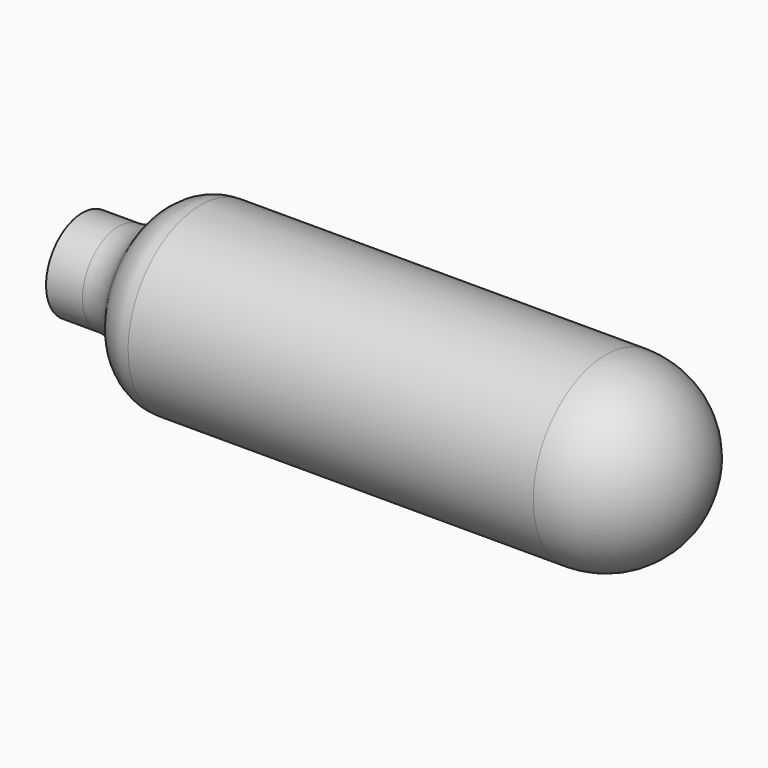
from build123d import *

# Parameters (mm, degrees)
F2_R = 9.525
F4_R = 5.08


# Not quite as in the source:
# - a fillet or chamfer that OpenCascade refuses, or shapes differently, is made with other operations: its cross-section is extruded or revolved along the edge and cut away or added


with BuildPart() as f1:
    # F0 (on Front) → F1 (revolve)
    with BuildSketch(Plane.XZ):
        Polygon((0, 4.7625), (0, 0), (64.516, 0), (64.516, 9.525), (8.89, 9.525), (8.89, 4.7625), align=None)
    revolve(axis=Axis((32.258, 0, 0), (1, 0, 0)))

    # F2
    f2_edges = [f1.edges().sort_by_distance(p)[0] for p in [
        (64.516, 0, -9.525),
    ]]
    fillet(f2_edges, radius=F2_R)

    # F3: fillet of radius 5.08 on 1 edges, made by hand

    # F3_s1 → F3_t2 (revolve)
    with BuildSketch(Plane.XZ):
        with BuildLine():
            ThreePointArc((8.89, 9.525), (7.2979698235, 6.1398455468), (3.8199315833, 4.7625))
            Line((3.8199315833, 4.7625), (8.89, 4.7625))
            Line((8.89, 4.7625), (8.89, 9.525))
        make_face()
    revolve(axis=Axis((8.89, 0, 0), (1, 0, 0)))

    # F4
    f4_edges = [f1.edges().sort_by_distance(p)[0] for p in [
        (8.89, 0, -9.525),
    ]]
    fillet(f4_edges, radius=F4_R)


solid = f1.part
